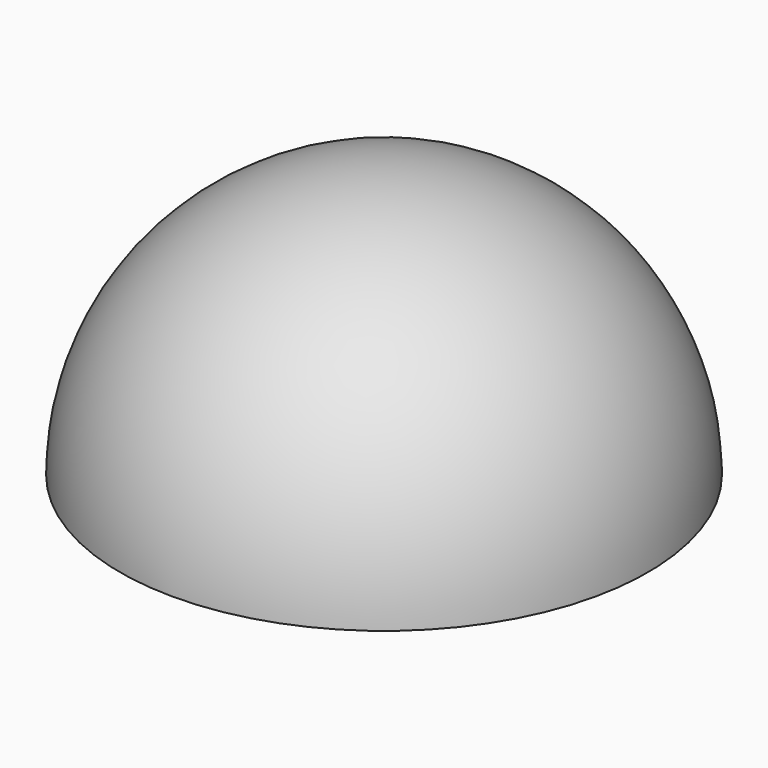
from build123d import *

# Parameters (mm, degrees)
F1_ANGLE = 180


# Not quite as in the source:
# - ends of sketch curves that miss each other by under 0.0002 mm in the source are joined


with BuildPart() as f1:
    # F0 (on Top) → F1 (revolve)
    with BuildSketch(Plane.XY):
        with BuildLine():
            ThreePointArc((0, -1.0028e-06), (38.1000010028, 38.1), (0, 76.2000010028))
            Line((0, 76.2000010028), (0, -1.0028e-06))
        make_face()
    revolve(axis=Axis((0, 38.1, 0), (0, -1, 0)), revolution_arc=F1_ANGLE)


solid = f1.part
